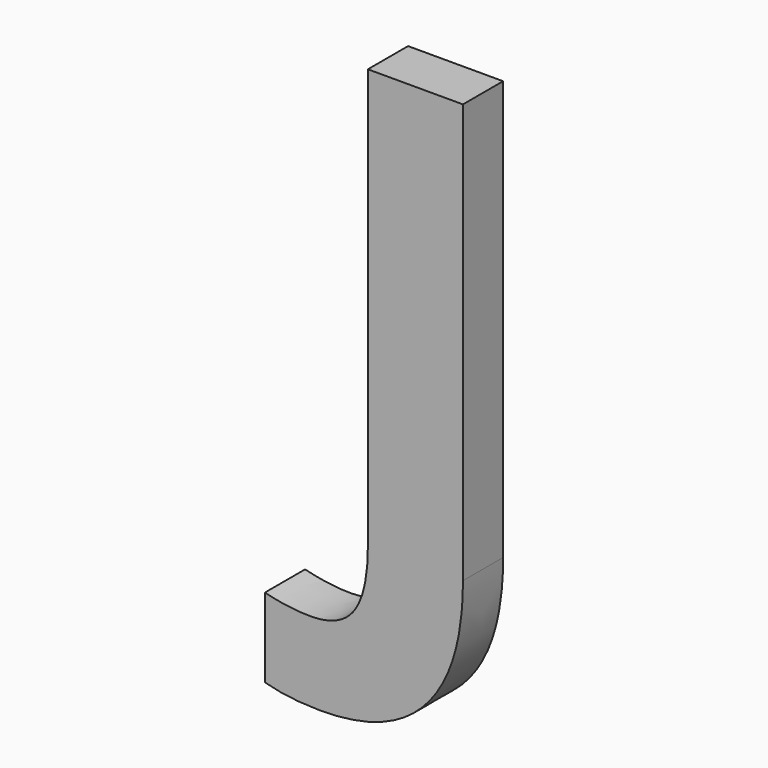
from build123d import *

# Parameters (mm, degrees)
F0_TEXT_SIZE = 62.5
F1_DEPTH     = 5


# Not quite as in the source:
# - Text() gives the source's letters only with a copy of the font that has no kerning and outlines rounded to 1/6400 em; it was checked with that copy


with BuildPart() as f1:
    # F0 (on Front) → F1 (new body)
    with BuildSketch(Plane.XZ):
        with Locations((-56.8718621043, 8.0276385128)):
            Text('J', F0_TEXT_SIZE, font='Open Sans', font_style=FontStyle.BOLD, text_align=(TextAlign.LEFT, TextAlign.BOTTOM))
    extrude(amount=F1_DEPTH)


solid = f1.part
